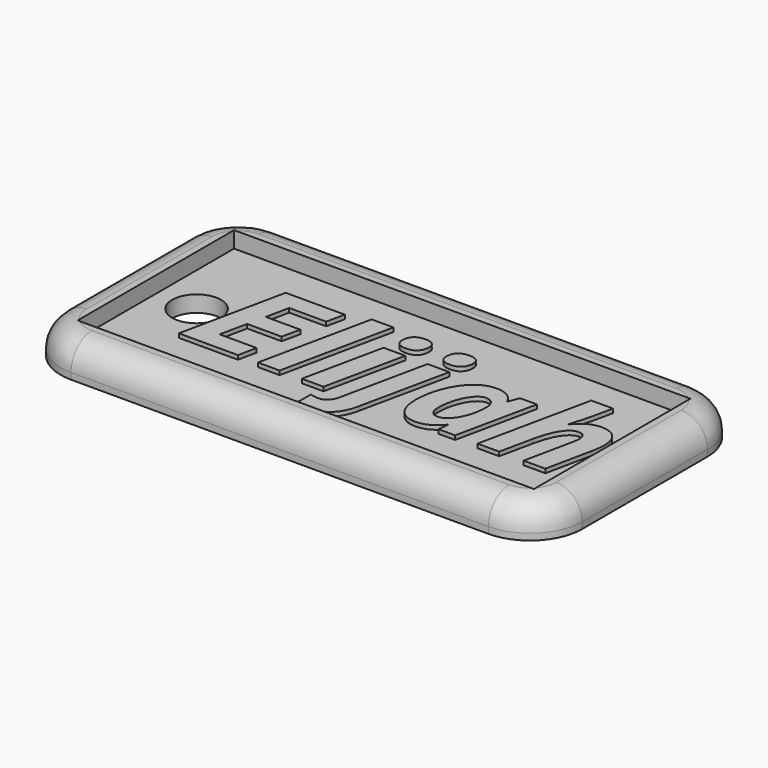
from build123d import *

# Parameters (mm, degrees)
F0_W         = 44.45
F0_H         = 19.05
F0_R         = 2.38125
F1_DEPTH     = 1.5875
F0_W_2       = 50.8
F0_H_2       = 25.4
F2_DEPTH     = 3.175
F3_R         = 5.08
F4_T1_DEPTH  = 40.64
F4_T3_DEPTH  = 15.24
F4_T6_ANGLE  = 90
F4_T8_ANGLE  = 90
F4_T10_ANGLE = 90
F4_T12_ANGLE = 90
F5_TEXT_SIZE = 14.404536862
F6_DEPTH     = 0.396875


# Not quite as in the source:
# - a fillet or chamfer that OpenCascade refuses, or shapes differently, is made with other operations: its cross-section is extruded or revolved along the edge and cut away or added
# - Text() gives the source's letters only with a copy of the font that has no kerning and outlines rounded to 1/6400 em; it was checked with that copy


with BuildPart() as f1:
    # F0 (on Top) → F1 (new body)
    with BuildSketch(Plane.XY):
        with Locations((25.4, 12.7)):
            Rectangle(F0_W, F0_H)
        with Locations((7.14375, 12.7)):
            Circle(F0_R, mode=Mode.SUBTRACT)
    extrude(amount=F1_DEPTH)

    # F0 (on Top) → F2 (join)
    with BuildSketch(Plane.XY):
        with Locations((25.4, 12.7)):
            Rectangle(F0_W_2, F0_H_2)
        with Locations((25.4, 12.7)):
            Rectangle(F0_W, F0_H, mode=Mode.SUBTRACT)
    extrude(amount=F2_DEPTH)

    # F3
    f3_edges = [f1.edges().sort_by_distance(p)[0] for p in [
        (50.8, 0, 1.5875),
        (50.8, 25.4, 1.5875),
        (0, 0, 1.5875),
        (0, 25.4, 1.5875),
    ]]
    fillet(f3_edges, radius=F3_R)

    # F4: fillet of radius 2.54 on 8 edges, made by hand

    # F4_s2 → F4_t1 (cut)
    with BuildSketch(Plane.YZ.offset(5.08)):
        with BuildLine():
            ThreePointArc((25.4, 0.635), (24.6560512242, 2.4310512242), (22.86, 3.175))
            Line((22.86, 3.175), (25.4, 3.175))
            Line((25.4, 3.175), (25.4, 0.635))
        make_face()
        with BuildLine():
            ThreePointArc((0, 0.635), (0.7439487758, 2.4310512242), (2.54, 3.175))
            Line((2.54, 3.175), (0, 3.175))
            Line((0, 3.175), (0, 0.635))
        make_face()
    extrude(amount=F4_T1_DEPTH, mode=Mode.SUBTRACT)

    # F4_s4 → F4_t3 (cut)
    with BuildSketch(Plane.XZ.offset(-20.32)):
        with BuildLine():
            ThreePointArc((0, 0.635), (0.7439487758, 2.4310512242), (2.54, 3.175))
            Line((2.54, 3.175), (0, 3.175))
            Line((0, 3.175), (0, 0.635))
        make_face()
        with BuildLine():
            ThreePointArc((50.8, 0.635), (50.0560512242, 2.4310512242), (48.26, 3.175))
            Line((48.26, 3.175), (50.8, 3.175))
            Line((50.8, 3.175), (50.8, 0.635))
        make_face()
    extrude(amount=F4_T3_DEPTH, mode=Mode.SUBTRACT)

    # F4_s5 → F4_t6 (revolve, cut)
    with BuildSketch(Plane.XZ.offset(-20.32)):
        with BuildLine():
            ThreePointArc((0, 0.635), (0.7439487758, 2.4310512242), (2.54, 3.175))
            Line((2.54, 3.175), (0, 3.175))
            Line((0, 3.175), (0, 0.635))
        make_face()
    revolve(axis=Axis((5.08, 20.32, 3.175), (0, 0, -1)), revolution_arc=F4_T6_ANGLE, mode=Mode.SUBTRACT)

    # F4_s7 → F4_t8 (revolve, cut)
    with BuildSketch(Plane.XZ.offset(-5.08)):
        with BuildLine():
            ThreePointArc((0, 0.635), (0.7439487758, 2.4310512242), (2.54, 3.175))
            Line((2.54, 3.175), (0, 3.175))
            Line((0, 3.175), (0, 0.635))
        make_face()
    revolve(axis=Axis((5.08, 5.08, 3.175), (0, 0, 1)), revolution_arc=F4_T8_ANGLE, mode=Mode.SUBTRACT)

    # F4_s9 → F4_t10 (revolve, cut)
    with BuildSketch(Plane.XZ.offset(-20.32)):
        with BuildLine():
            ThreePointArc((50.8, 0.635), (50.0560512242, 2.4310512242), (48.26, 3.175))
            Line((48.26, 3.175), (50.8, 3.175))
            Line((50.8, 3.175), (50.8, 0.635))
        make_face()
    revolve(axis=Axis((45.72, 20.32, 3.175), (0, 0, 1)), revolution_arc=F4_T10_ANGLE, mode=Mode.SUBTRACT)

    # F4_s11 → F4_t12 (revolve, cut)
    with BuildSketch(Plane.YZ.offset(45.72)):
        with BuildLine():
            ThreePointArc((0, 0.635), (0.7439487758, 2.4310512242), (2.54, 3.175))
            Line((2.54, 3.175), (0, 3.175))
            Line((0, 3.175), (0, 0.635))
        make_face()
    revolve(axis=Axis((45.72, 5.08, 3.175), (0, 0, 1)), revolution_arc=F4_T12_ANGLE, mode=Mode.SUBTRACT)

    # F5 (on face) → F6 (join)
    with BuildSketch(Plane.XY.offset(1.5875)):
        with Locations((8.7156806253, 8.1183684362)):
            Text('Elijah', F5_TEXT_SIZE, font='Open Sans', font_style=FontStyle.BOLDITALIC, text_align=(TextAlign.LEFT, TextAlign.BOTTOM))
    extrude(amount=F6_DEPTH)


solid = f1.part
